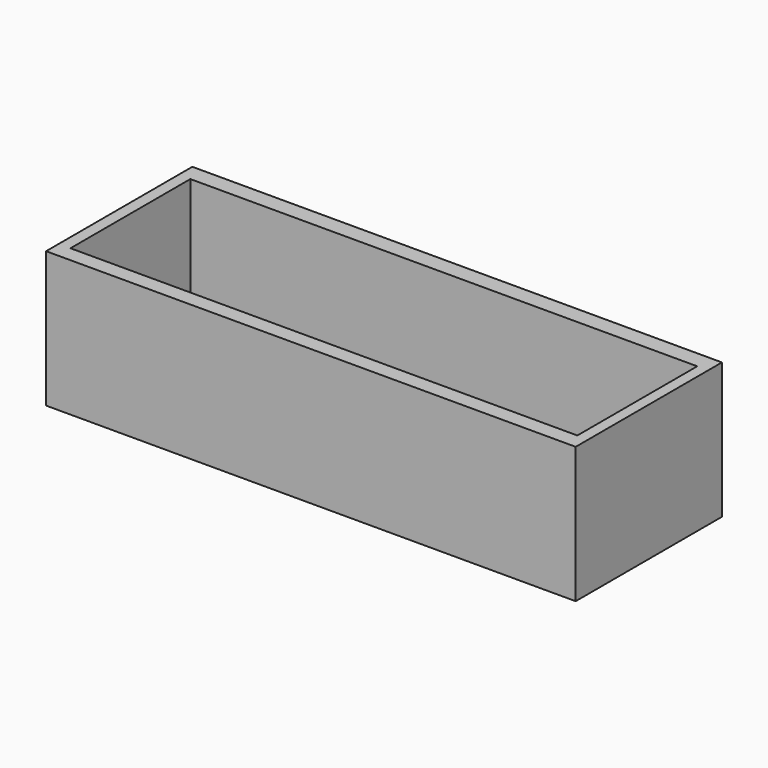
from build123d import *

# Parameters (mm, degrees)
F0_W     = 98.960949108
F0_H     = 34.1609604657
F0_W_2   = 94.7147086263
F0_H_2   = 27.9996693134
F1_DEPTH = 25.4


# Not quite as in the source:
# - a feature names something its author has since deleted; it is built from what else it names


with BuildPart() as f1:
    # F0 (on Top) → F1 (new body)
    with BuildSketch(Plane.XY):
        with Locations((-27.005889453, 1.987118274)):
            Rectangle(F0_W, F0_H)
        with Locations((-26.931297034, 1.8579196185)):
            Rectangle(F0_W_2, F0_H_2, mode=Mode.SUBTRACT)
    extrude(amount=F1_DEPTH)


solid = f1.part
